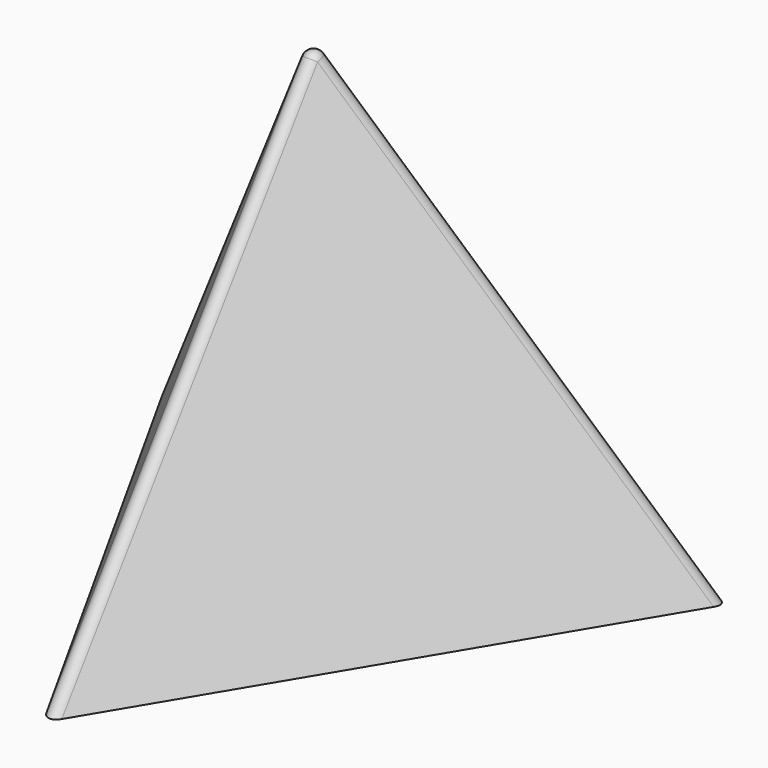
from build123d import *

# Parameters (mm, degrees)
F1_DEPTH     = 0.0254
F5_T1_DEPTH  = 77.4636340451
F5_T3_DEPTH  = 77.4636340451
F5_T5_DEPTH  = 77.4636340451
F5_T7_DEPTH  = 81.7261129419
F5_T9_DEPTH  = 81.7261129419
F5_T11_DEPTH = 81.7261129419
F5_T16_DEPTH = 4.7473188038


# Not quite as in the source:
# - a fillet or chamfer that OpenCascade refuses, or shapes differently, is made with other operations: its cross-section is extruded or revolved along the edge and cut away or added


with BuildPart() as f1:
    # F0 (on Top) → F1 (new body)
    with BuildSketch(Plane.XY):
        Polygon((-37.7498417943, 22.5926856417), (-0.6909188082, -43.9886648036), (38.4407606026, 21.3959791619), align=None)
    extrude(amount=F1_DEPTH)

    # F1_face (on face) → F4 section 0
    with BuildSketch(Plane.XY.offset(0.0254), mode=Mode.PRIVATE) as f4_s0:
        Polygon((38.4407606026, 21.3959791619), (-37.7498417943, 22.5926856417), (-0.6909188082, -43.9886648036), align=None)
    loft([f4_s0.sketch, Vertex(0, 0, 63.5)])

    # F5: fillet of radius 1.27 on 6 edges, made by hand

    # F5_s2 → F5_t1 (cut)
    with BuildSketch(Plane(origin=(-18.8367378497, 33.8427386163, 0), x_dir=(0, 0, 1), z_dir=(0.486337572, -0.8737710032, 0))):
        with BuildLine():
            ThreePointArc((0.0254, 21.9970452561), (0.0063659549, 21.8713184471), (0, 21.7443184471))
            Line((0, 21.7443184471), (0, 21.9970452561))
            Line((0, 21.9970452561), (0.0254, 21.9970452561))
        make_face()
    extrude(amount=F5_T1_DEPTH, mode=Mode.SUBTRACT)

    # F5_s4 → F5_t3 (cut)
    with BuildSketch(Plane(origin=(-19.8903024505, -33.2344628104, 0), x_dir=(0, 0, 1), z_dir=(0.5135390999, 0.8580661938, 0))):
        with BuildLine():
            ThreePointArc((0.0254, 21.9970452561), (0.0063659549, 21.8713184471), (0, 21.7443184471))
            Line((0, 21.7443184471), (0, 21.9970452561))
            Line((0, 21.9970452561), (0.0254, 21.9970452561))
        make_face()
    extrude(amount=F5_T3_DEPTH, mode=Mode.SUBTRACT)

    # F5_s6 → F5_t5 (cut)
    with BuildSketch(Plane(origin=(38.7270403002, -0.6082758058, 0), x_dir=(0, 0, 1), z_dir=(-0.9998766719, 0.0157048094, 0))):
        with BuildLine():
            ThreePointArc((0.0254, 21.9970452561), (0.0063659549, 21.8713184471), (0, 21.7443184471))
            Line((0, 21.7443184471), (0, 21.9970452561))
            Line((0, 21.9970452561), (0.0254, 21.9970452561))
        make_face()
    extrude(amount=F5_T5_DEPTH, mode=Mode.SUBTRACT)

    # F5_s8 → F5_t7 (cut)
    with BuildSketch(Plane(origin=(-15.9953348191, 9.5729559152, -26.8954101859), x_dir=(0.5135390999, 0.8580661938, 0), z_dir=(0.4887963318, -0.2925369046, 0.8218882561))):
        with BuildLine():
            ThreePointArc((1.0392181385, 34.6933141222), (0, 35.2332965467), (-1.0392181385, 34.6933141222))
            Line((-1.0392181385, 34.6933141222), (0, 36.172695408))
            Line((0, 36.172695408), (1.0392181385, 34.6933141222))
        make_face()
    extrude(amount=F5_T7_DEPTH, mode=Mode.SUBTRACT)

    # F5_s10 → F5_t9 (cut)
    with BuildSketch(Plane(origin=(16.2880904214, 9.0658883378, -26.8954101859), x_dir=(0.486337572, -0.8737710032, 0), z_dir=(-0.4977425568, -0.2770415883, 0.8218882561))):
        with BuildLine():
            ThreePointArc((-1.0392181385, 34.6933141222), (0, 35.2332965467), (1.0392181385, 34.6933141222))
            Line((1.0392181385, 34.6933141222), (0, 36.172695408))
            Line((0, 36.172695408), (-1.0392181385, 34.6933141222))
        make_face()
    extrude(amount=F5_T9_DEPTH, mode=Mode.SUBTRACT)

    # F5_s12 → F5_t11 (cut)
    with BuildSketch(Plane(origin=(-0.2927556023, -18.638844253, -26.8954101859), x_dir=(-0.9998766719, 0.0157048094, 0), z_dir=(0.008946225, 0.5695784929, 0.8218882561))):
        with BuildLine():
            ThreePointArc((-1.0392181385, 34.6933141222), (0, 35.2332965467), (1.0392181385, 34.6933141222))
            Line((1.0392181385, 34.6933141222), (0, 36.172695408))
            Line((0, 36.172695408), (-1.0392181385, 34.6933141222))
        make_face()
    extrude(amount=F5_T11_DEPTH, mode=Mode.SUBTRACT)


with BuildPart() as f5_tool14:
    # F5_s15 → F5_t16 (new body)
    with BuildSketch(Plane.XY.offset(59.6214715655)):
        Polygon((4.8212890631, 4.6721775887), (-4.6721775887, 4.8212890631), (-4.8212890631, -4.6721775887), (4.6721775887, -4.8212890631), align=None)
    extrude(amount=F5_T16_DEPTH)

    split(bisect_by=Plane(origin=(-24.3904739903, -13.5756437975, 40.2743222578), x_dir=(0.486337572, -0.8737710032, 0), z_dir=(-0.4977425568, -0.2770415883, 0.8218882561)), keep=Keep.TOP)

    split(bisect_by=Plane(origin=(0.4383845938, 27.9105919847, 40.2743222578), x_dir=(-0.9998766719, 0.0157048094, 0), z_dir=(0.008946225, 0.5695784929, 0.8218882561)), keep=Keep.TOP)

    split(bisect_by=Plane(origin=(23.9520893965, -14.3349481872, 40.2743222578), x_dir=(0.5135390999, 0.8580661938, 0), z_dir=(0.4887963318, -0.2925369046, 0.8218882561)), keep=Keep.TOP)

    split(bisect_by=Plane(origin=(0.3089197728, 19.6679670247, 6.8167506947), x_dir=(0.9998766719, -0.0157048094, 0), z_dir=(-0.0148390137, -0.9447541355, -0.3274437771)), keep=Keep.TOP)

    split(bisect_by=Plane(origin=(16.8784991978, -10.1015158833, 6.8167506947), x_dir=(-0.5135390999, -0.8580661938, 0), z_dir=(-0.8107615748, 0.4852280306, -0.3274437771)), keep=Keep.TOP)

    split(bisect_by=Plane(origin=(-17.1874189706, -9.5664511414, 6.8167506947), x_dir=(-0.486337572, 0.8737710032, 0), z_dir=(0.8256005885, 0.4595261049, -0.3274437771)), keep=Keep.TOP)

    # F5_s23 → F5_t24 (revolve, cut)
    with BuildSketch(Plane(origin=(0, 0, 59.6214715655), x_dir=(0, 0, -1), z_dir=(0.0157048094, 0.9998766719, 0))):
        with BuildLine():
            ThreePointArc((0, -1.27), (1.27, 0), (0, 1.27))
            Line((0, 1.27), (0, -1.27))
        make_face()
    revolve(axis=Axis((0, 0, 59.6214715655), (-0.9998766719, 0.0157048094, 0)), mode=Mode.SUBTRACT)


with BuildPart() as f1_1:
    add(f1.part)

    # F5_t13: cut F5_tool14
    add(f5_tool14.part, mode=Mode.SUBTRACT)


solid = f1_1.part
